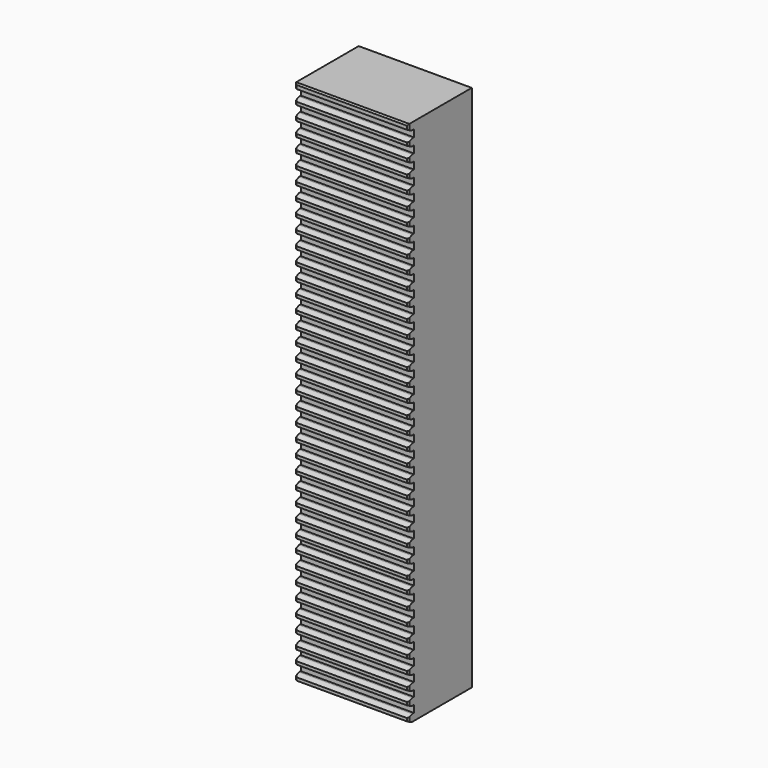
from build123d import *

# Parameters (mm, degrees)
F0_W         = 40.64
F0_H         = 35.56
F1_DEPTH     = 190.5
F2_W         = 2.54
F2_H         = 2.54
F2_H_2       = 2.1528191495
F2_H_3       = 2.1739019747
F3_DEPTH     = 40.641
F4_DEPTH     = 5.08
F5_DEPTH     = 1.905
F6_SIZE      = 0.508
F7_W         = 40.64
F7_H         = 0.7532788758
F8_DEPTH     = 28.576
F9_SIZE      = 0.508
F10_T1_DEPTH = 47.225382798


# Not quite as in the source:
# - a fillet or chamfer that OpenCascade refuses, or shapes differently, is made with other operations: its cross-section is extruded or revolved along the edge and cut away or added


with BuildPart() as f1:
    # F0 (on Top) → F1 (new body)
    with BuildSketch(Plane.XY):
        with Locations((20.32, 17.78)):
            Rectangle(F0_W, F0_H)
    extrude(amount=F1_DEPTH)

    # F2 (on face) → F3 (cut, through all)
    with BuildSketch(Plane(origin=(0, 0, 0), x_dir=(0, -1, 0), z_dir=(-1, 0, 0))):
        with Locations((-1.27, 186.69)):
            Rectangle(F2_W, F2_H)
        with Locations((-1.27, 181.61)):
            Rectangle(F2_W, F2_H)
        with Locations((-1.27, 176.53)):
            Rectangle(F2_W, F2_H)
        with Locations((-1.27, 171.45)):
            Rectangle(F2_W, F2_H)
        with Locations((-1.27, 166.37)):
            Rectangle(F2_W, F2_H)
        with Locations((-1.27, 161.29)):
            Rectangle(F2_W, F2_H)
        with Locations((-1.27, 156.21)):
            Rectangle(F2_W, F2_H)
        with Locations((-1.27, 151.13)):
            Rectangle(F2_W, F2_H)
        with Locations((-1.27, 146.05)):
            Rectangle(F2_W, F2_H)
        with Locations((-1.27, 140.97)):
            Rectangle(F2_W, F2_H)
        with Locations((-1.27, 135.89)):
            Rectangle(F2_W, F2_H)
        with Locations((-1.27, 130.81)):
            Rectangle(F2_W, F2_H)
        with Locations((-1.27, 125.73)):
            Rectangle(F2_W, F2_H)
        with Locations((-1.27, 120.65)):
            Rectangle(F2_W, F2_H)
        with Locations((-1.27, 115.57)):
            Rectangle(F2_W, F2_H)
        with Locations((-1.27, 110.49)):
            Rectangle(F2_W, F2_H)
        with Locations((-1.27, 105.41)):
            Rectangle(F2_W, F2_H)
        with Locations((-1.27, 100.33)):
            Rectangle(F2_W, F2_H)
        with Locations((-1.27, 95.25)):
            Rectangle(F2_W, F2_H)
        with Locations((-1.27, 90.17)):
            Rectangle(F2_W, F2_H)
        with Locations((-1.27, 85.09)):
            Rectangle(F2_W, F2_H)
        with Locations((-1.27, 80.01)):
            Rectangle(F2_W, F2_H)
        with Locations((-1.27, 74.93)):
            Rectangle(F2_W, F2_H)
        with Locations((-1.27, 69.85)):
            Rectangle(F2_W, F2_H)
        with Locations((-1.27, 64.77)):
            Rectangle(F2_W, F2_H)
        with Locations((-1.27, 59.69)):
            Rectangle(F2_W, F2_H)
        with Locations((-1.27, 54.61)):
            Rectangle(F2_W, F2_H)
        with Locations((-1.27, 49.53)):
            Rectangle(F2_W, F2_H)
        with Locations((-1.27, 44.6435904253)):
            Rectangle(F2_W, F2_H_2)
        with Locations((-1.27, 39.7571808505)):
            Rectangle(F2_W, F2_H)
        with Locations((-1.27, 34.6771808505)):
            Rectangle(F2_W, F2_H)
        with Locations((-1.27, 29.5971808505)):
            Rectangle(F2_W, F2_H)
        with Locations((-1.27, 24.5171808505)):
            Rectangle(F2_W, F2_H)
        with Locations((-1.27, 19.4371808505)):
            Rectangle(F2_W, F2_H)
        with Locations((-1.27, 14.3571808505)):
            Rectangle(F2_W, F2_H)
        with Locations((-1.27, 9.4602298632)):
            Rectangle(F2_W, F2_H_3)
        with Locations((-1.27, 4.5632788758)):
            Rectangle(F2_W, F2_H)
    extrude(amount=-F3_DEPTH, mode=Mode.SUBTRACT)

    # F4 (cut): a face of the model
    f4_faces = [f1.faces().sort_by_distance(p)[0] for p in [
        (20.32, 35.56, 95.25),
    ]]
    extrude(f4_faces, amount=-F4_DEPTH, mode=Mode.SUBTRACT)

    # F5 (cut): a face of the model
    f5_faces = [f1.faces().sort_by_distance(p)[0] for p in [
        (20.32, 30.48, 95.25),
    ]]
    extrude(f5_faces, amount=-F5_DEPTH, mode=Mode.SUBTRACT)

    # F6
    f6_edges = [f1.edges().sort_by_distance(p)[0] for p in [
        (20.32, 0, 190.5),
        (20.32, 0, 187.96),
        (20.32, 0, 185.42),
        (20.32, 0, 182.88),
        (20.32, 0, 180.34),
        (20.32, 0, 177.8),
        (40.64, 0, 189.23),
        (0, 0, 189.23),
        (40.64, 0, 184.15),
        (0, 0, 184.15),
        (40.64, 0, 179.07),
        (0, 0, 179.07),
        (20.32, 0, 172.72),
        (40.64, 0, 173.99),
        (20.32, 0, 175.26),
        (0, 0, 173.99),
        (20.32, 0, 167.64),
        (40.64, 0, 168.91),
        (20.32, 0, 170.18),
        (0, 0, 168.91),
        (20.32, 0, 162.56),
        (40.64, 0, 163.83),
        (20.32, 0, 165.1),
        (0, 0, 163.83),
        (20.32, 0, 157.48),
        (40.64, 0, 158.75),
        (20.32, 0, 160.02),
        (0, 0, 158.75),
        (20.32, 0, 152.4),
        (40.64, 0, 153.67),
        (20.32, 0, 154.94),
        (0, 0, 153.67),
        (20.32, 0, 147.32),
        (40.64, 0, 148.59),
        (20.32, 0, 149.86),
        (0, 0, 148.59),
        (20.32, 0, 142.24),
        (40.64, 0, 143.51),
        (20.32, 0, 144.78),
        (0, 0, 143.51),
        (20.32, 0, 137.16),
        (40.64, 0, 138.43),
        (20.32, 0, 139.7),
        (0, 0, 138.43),
        (20.32, 0, 132.08),
        (40.64, 0, 133.35),
        (20.32, 0, 134.62),
        (0, 0, 133.35),
        (20.32, 0, 127),
        (40.64, 0, 128.27),
        (20.32, 0, 129.54),
        (0, 0, 128.27),
        (20.32, 0, 121.92),
        (40.64, 0, 123.19),
        (20.32, 0, 124.46),
        (0, 0, 123.19),
        (20.32, 0, 116.84),
        (40.64, 0, 118.11),
        (20.32, 0, 119.38),
        (0, 0, 118.11),
        (20.32, 0, 111.76),
        (40.64, 0, 113.03),
        (20.32, 0, 114.3),
        (0, 0, 113.03),
        (20.32, 0, 106.68),
        (40.64, 0, 107.95),
        (20.32, 0, 109.22),
        (0, 0, 107.95),
        (20.32, 0, 101.6),
        (40.64, 0, 102.87),
        (20.32, 0, 104.14),
        (0, 0, 102.87),
        (20.32, 0, 96.52),
        (40.64, 0, 97.79),
        (20.32, 0, 99.06),
        (0, 0, 97.79),
        (20.32, 0, 91.44),
        (40.64, 0, 92.71),
        (20.32, 0, 93.98),
        (0, 0, 92.71),
        (20.32, 0, 86.36),
        (40.64, 0, 87.63),
        (20.32, 0, 88.9),
        (0, 0, 87.63),
        (20.32, 0, 81.28),
        (40.64, 0, 82.55),
        (20.32, 0, 83.82),
        (0, 0, 82.55),
        (20.32, 0, 76.2),
        (40.64, 0, 77.47),
        (20.32, 0, 78.74),
        (0, 0, 77.47),
        (20.32, 0, 73.66),
        (20.32, 0, 71.12),
        (40.64, 0, 72.39),
        (0, 0, 72.39),
        (20.32, 0, 66.04),
        (40.64, 0, 67.31),
        (20.32, 0, 68.58),
        (0, 0, 67.31),
        (20.32, 0, 60.96),
        (40.64, 0, 62.23),
        (20.32, 0, 63.5),
        (0, 0, 62.23),
        (20.32, 0, 55.88),
        (40.64, 0, 57.15),
        (20.32, 0, 58.42),
        (0, 0, 57.15),
        (20.32, 0, 50.8),
        (40.64, 0, 52.07),
        (20.32, 0, 53.34),
        (0, 0, 52.07),
        (20.32, 0, 45.72),
        (40.64, 0, 46.99),
        (20.32, 0, 48.26),
        (0, 0, 46.99),
        (20.32, 0, 41.027181),
        (40.64, 0, 42.297181),
        (20.32, 0, 43.567181),
        (0, 0, 42.297181),
        (20.32, 0, 35.947181),
        (40.64, 0, 37.217181),
        (20.32, 0, 38.487181),
        (0, 0, 37.217181),
        (20.32, 0, 30.867181),
        (40.64, 0, 32.137181),
        (20.32, 0, 33.407181),
        (0, 0, 32.137181),
        (20.32, 0, 25.787181),
        (40.64, 0, 27.057181),
        (20.32, 0, 28.327181),
        (0, 0, 27.057181),
        (20.32, 0, 20.707181),
        (40.64, 0, 21.977181),
        (20.32, 0, 23.247181),
        (0, 0, 21.977181),
        (20.32, 0, 15.627181),
        (40.64, 0, 16.897181),
        (20.32, 0, 18.167181),
        (0, 0, 16.897181),
        (20.32, 0, 10.547181),
        (40.64, 0, 11.817181),
        (20.32, 0, 13.087181),
        (0, 0, 11.817181),
        (20.32, 0, 5.833279),
        (40.64, 0, 7.103279),
        (20.32, 0, 8.373279),
        (0, 0, 7.103279),
    ]]
    chamfer(f6_edges, length=F6_SIZE)

    # F7 (on face) → F8 (cut, through all)
    with BuildSketch(Plane.XZ):
        with Locations((20.32, 0.3766394379)):
            Rectangle(F7_W, F7_H)
    extrude(amount=-F8_DEPTH, mode=Mode.SUBTRACT)

    # F9
    f9_edges = [f1.edges().sort_by_distance(p)[0] for p in [
        (20.32, 0, 0.753279),
        (40.64, 0, 2.023279),
        (20.32, 0, 3.293279),
        (0, 0, 2.023279),
    ]]
    chamfer(f9_edges, length=F9_SIZE)

    # F10: chamfer of 1.27 on 75 edges, made by hand

    # F10_s2 → F10_t1 (cut)
    with BuildSketch(Plane.YZ.offset(-3.292691399)):
        Polygon((1.778, 187.96), (-0.3900256121, 188.8580256121), (0.508, 187.96), align=None)
        Polygon((1.778, 185.42), (-0.3900256121, 184.5219743879), (0.508, 185.42), align=None)
        Polygon((1.778, 182.88), (-0.3900256121, 183.7780256121), (0.508, 182.88), align=None)
        Polygon((1.778, 180.34), (-0.3900256121, 179.4419743879), (0.508, 180.34), align=None)
        Polygon((1.778, 177.8), (-0.3900256121, 178.6980256121), (0.508, 177.8), align=None)
        Polygon((1.778, 172.72), (-0.3900256121, 173.6180256121), (0.508, 172.72), align=None)
        Polygon((1.778, 170.18), (-0.3900256121, 169.2819743879), (0.508, 170.18), align=None)
        Polygon((1.778, 167.64), (-0.3900256121, 168.5380256121), (0.508, 167.64), align=None)
        Polygon((1.778, 165.1), (-0.3900256121, 164.2019743879), (0.508, 165.1), align=None)
        Polygon((1.778, 162.56), (-0.3900256121, 163.4580256121), (0.508, 162.56), align=None)
        Polygon((1.778, 160.02), (-0.3900256121, 159.1219743879), (0.508, 160.02), align=None)
        Polygon((1.778, 157.48), (-0.3900256121, 158.3780256121), (0.508, 157.48), align=None)
        Polygon((1.778, 154.94), (-0.3900256121, 154.0419743879), (0.508, 154.94), align=None)
        Polygon((1.778, 152.4), (-0.3900256121, 153.2980256121), (0.508, 152.4), align=None)
        Polygon((1.778, 149.86), (-0.3900256121, 148.9619743879), (0.508, 149.86), align=None)
        Polygon((1.778, 147.32), (-0.3900256121, 148.2180256121), (0.508, 147.32), align=None)
        Polygon((1.778, 144.78), (-0.3900256121, 143.8819743879), (0.508, 144.78), align=None)
        Polygon((1.778, 137.16), (-0.3900256121, 138.0580256121), (0.508, 137.16), align=None)
        Polygon((1.778, 139.7), (-0.3900256121, 138.8019743879), (0.508, 139.7), align=None)
        Polygon((1.778, 134.62), (-0.3900256121, 133.7219743879), (0.508, 134.62), align=None)
        Polygon((1.778, 132.08), (-0.3900256121, 132.9780256121), (0.508, 132.08), align=None)
        Polygon((1.778, 129.54), (-0.3900256121, 128.6419743879), (0.508, 129.54), align=None)
        Polygon((1.778, 127), (-0.3900256121, 127.8980256121), (0.508, 127), align=None)
        Polygon((1.778, 124.46), (-0.3900256121, 123.5619743879), (0.508, 124.46), align=None)
        Polygon((1.778, 121.92), (-0.3900256121, 122.8180256121), (0.508, 121.92), align=None)
        Polygon((1.778, 119.38), (-0.3900256121, 118.4819743879), (0.508, 119.38), align=None)
        Polygon((1.778, 116.84), (-0.3900256121, 117.7380256121), (0.508, 116.84), align=None)
        Polygon((1.778, 114.3), (-0.3900256121, 113.4019743879), (0.508, 114.3), align=None)
        Polygon((1.778, 111.76), (-0.3900256121, 112.6580256121), (0.508, 111.76), align=None)
        Polygon((1.778, 109.22), (-0.3900256121, 108.3219743879), (0.508, 109.22), align=None)
        Polygon((1.778, 106.68), (-0.3900256121, 107.5780256121), (0.508, 106.68), align=None)
        Polygon((1.778, 104.14), (-0.3900256121, 103.2419743879), (0.508, 104.14), align=None)
        Polygon((1.778, 101.6), (-0.3900256121, 102.4980256121), (0.508, 101.6), align=None)
        Polygon((1.778, 99.06), (-0.3900256121, 98.1619743879), (0.508, 99.06), align=None)
        Polygon((1.778, 96.52), (-0.3900256121, 97.4180256121), (0.508, 96.52), align=None)
        Polygon((1.778, 93.98), (-0.3900256121, 93.0819743879), (0.508, 93.98), align=None)
        Polygon((1.778, 91.44), (-0.3900256121, 92.3380256121), (0.508, 91.44), align=None)
        Polygon((1.778, 88.9), (-0.3900256121, 88.0019743879), (0.508, 88.9), align=None)
        Polygon((1.778, 86.36), (-0.3900256121, 87.2580256121), (0.508, 86.36), align=None)
        Polygon((1.778, 83.82), (-0.3900256121, 82.9219743879), (0.508, 83.82), align=None)
        Polygon((1.778, 81.28), (-0.3900256121, 82.1780256121), (0.508, 81.28), align=None)
        Polygon((1.778, 78.74), (-0.3900256121, 77.8419743879), (0.508, 78.74), align=None)
        Polygon((1.778, 76.2), (-0.3900256121, 77.0980256121), (0.508, 76.2), align=None)
        Polygon((1.778, 73.66), (-0.3900256121, 72.7619743879), (0.508, 73.66), align=None)
        Polygon((1.778, 71.12), (-0.3900256121, 72.0180256121), (0.508, 71.12), align=None)
        Polygon((1.778, 68.58), (-0.3900256121, 67.6819743879), (0.508, 68.58), align=None)
        Polygon((1.778, 66.04), (-0.3900256121, 66.9380256121), (0.508, 66.04), align=None)
        Polygon((1.778, 63.5), (-0.3900256121, 62.6019743879), (0.508, 63.5), align=None)
        Polygon((1.778, 60.96), (-0.3900256121, 61.8580256121), (0.508, 60.96), align=None)
        Polygon((1.778, 55.88), (-0.3900256121, 56.7780256121), (0.508, 55.88), align=None)
        Polygon((1.778, 58.42), (-0.3900256121, 57.5219743879), (0.508, 58.42), align=None)
        Polygon((1.778, 53.34), (-0.3900256121, 52.4419743879), (0.508, 53.34), align=None)
        Polygon((1.778, 50.8), (-0.3900256121, 51.6980256121), (0.508, 50.8), align=None)
        Polygon((1.778, 48.26), (-0.3900256121, 47.3619743879), (0.508, 48.26), align=None)
        Polygon((1.778, 45.72), (-0.3900256121, 46.6180256121), (0.508, 45.72), align=None)
        Polygon((1.778, 35.9471808505), (-0.3900256121, 36.8452064626), (0.508, 35.9471808505), align=None)
        Polygon((1.778, 38.4871808505), (-0.3900256121, 37.5891552384), (0.508, 38.4871808505), align=None)
        Polygon((1.778, 33.4071808505), (-0.3900256121, 32.5091552384), (0.508, 33.4071808505), align=None)
        Polygon((1.778, 30.8671808505), (-0.3900256121, 31.7652064626), (0.508, 30.8671808505), align=None)
        Polygon((1.778, 41.0271808505), (-0.3900256121, 41.9252064626), (0.508, 41.0271808505), align=None)
        Polygon((1.778, 43.5671808505), (-0.3900256121, 42.6691552384), (0.508, 43.5671808505), align=None)
        Polygon((1.778, 28.3271808505), (-0.3900256121, 27.4291552384), (0.508, 28.3271808505), align=None)
        Polygon((1.778, 25.7871808505), (-0.3900256121, 26.6852064626), (0.508, 25.7871808505), align=None)
        Polygon((1.778, 15.6271808505), (-0.3900256121, 16.5252064626), (0.508, 15.6271808505), align=None)
        Polygon((1.778, 18.1671808505), (-0.3900256121, 17.2691552384), (0.508, 18.1671808505), align=None)
        Polygon((1.778, 13.0871808505), (-0.3900256121, 12.1891552384), (0.508, 13.0871808505), align=None)
        Polygon((1.778, 10.5471808505), (-0.3900256121, 11.4452064626), (0.508, 10.5471808505), align=None)
        Polygon((1.778, 5.8332788758), (-0.3900256121, 6.7313044879), (0.508, 5.8332788758), align=None)
        Polygon((1.778, 8.3732788758), (-0.3900256121, 7.4752532637), (0.508, 8.3732788758), align=None)
        Polygon((1.778, 3.2932788758), (-0.3900256121, 2.3952532637), (0.508, 3.2932788758), align=None)
        Polygon((1.778, 0.7532788758), (-0.3900256121, 1.6513044879), (0.508, 0.7532788758), align=None)
        Polygon((1.778, 20.7071808505), (-0.3900256121, 21.6052064626), (0.508, 20.7071808505), align=None)
        Polygon((1.778, 23.2471808505), (-0.3900256121, 22.3491552384), (0.508, 23.2471808505), align=None)
        Polygon((1.778, 175.26), (-0.3900256121, 174.3619743879), (0.508, 175.26), align=None)
        Polygon((1.778, 142.24), (-0.3900256121, 143.1380256121), (0.508, 142.24), align=None)
    extrude(amount=F10_T1_DEPTH, mode=Mode.SUBTRACT)


solid = f1.part
